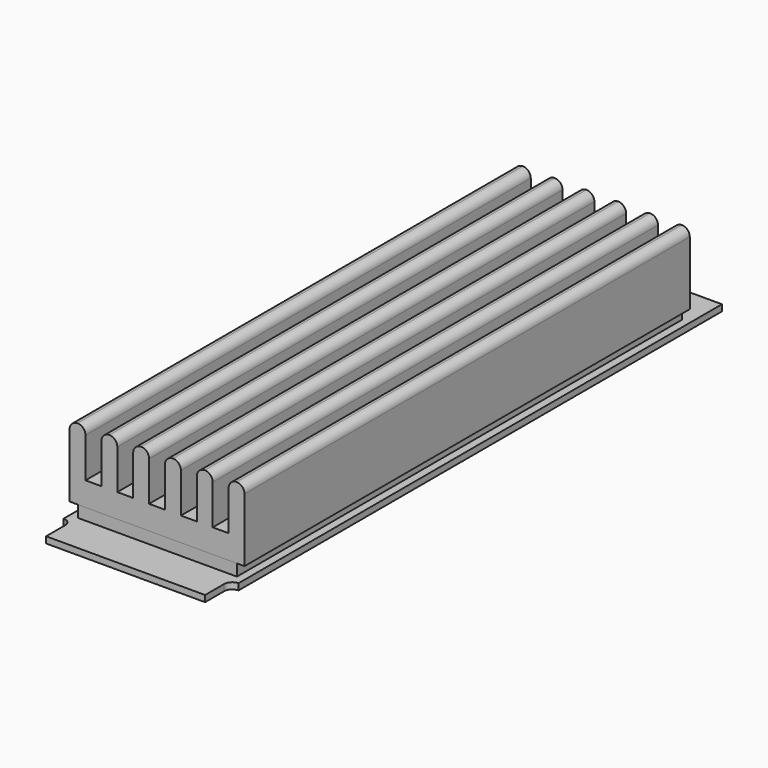
from build123d import *

# Parameters (mm, degrees)
F1_DEPTH = 0.8
F2_R     = 0.99999
F3_W     = 20
F3_H     = 70
F4_DEPTH = 1.5
F6_DEPTH = 0.801
F7_DEPTH = 0.1
F8_W     = 1
F8_H     = 2
F8_W_2   = 2
F8_H_2   = 6
F9_DEPTH = 35
F10_R    = 0.99999


# Not quite as in the source:
# - a fillet or chamfer is up to 0.001 mm smaller than in the source, because OpenCascade refuses the exact size


with BuildPart() as f1:
    # F0 (on Top) → F1 (new body)
    with BuildSketch(Plane.XY):
        Polygon((10.6782857925, 40.0528391576), (-11.3217142075, 40.0528391576), (-11.3217142075, -35.9471608424), (-10.3217142075, -35.9471608424), (-10.3217142075, -39.9471608424), (9.6782857925, -39.9471608424), (9.6782857925, -35.9471608424), (10.6782857925, -35.9471608424), align=None)
    extrude(amount=F1_DEPTH)

    # F2 (radius 1 in the source; OpenCascade refuses exactly that, so slightly less here)
    f2_edges = [f1.edges().sort_by_distance(p)[0] for p in [
        (9.678286, -35.947161, 0.4),
        (-10.321714, -35.947161, 0.4),
    ]]
    fillet(f2_edges, radius=F2_R)

    # F3 (on face) → F4 (join)
    with BuildSketch(Plane.XY.offset(0.8)):
        with Locations((-0.3217142075, 0.0528391576)):
            Rectangle(F3_W, F3_H)
    extrude(amount=F4_DEPTH)

    # F5 (on face) → F6 (cut, through all)
    with BuildSketch(Plane.XY.offset(0.8)):
        with BuildLine():
            ThreePointArc((-1.8217142075, 40.0528391576), (-0.3217142075, 38.5528391576), (1.1782857925, 40.0528391576))
            Line((1.1782857925, 40.0528391576), (-1.8217142075, 40.0528391576))
        make_face()
    extrude(amount=-F6_DEPTH, mode=Mode.SUBTRACT)

    # F5 (on face) → F7 (join)
    with BuildSketch(Plane.XY.offset(0.8)):
        with BuildLine():
            Line((2.4282857925, 40.0528391576), (1.1782857925, 40.0528391576))
            ThreePointArc((1.1782857925, 40.0528391576), (-0.3217142075, 38.5528391576), (-1.8217142075, 40.0528391576))
            Line((-1.8217142075, 40.0528391576), (-3.0717142075, 40.0528391576))
            ThreePointArc((-3.0717142075, 40.0528391576), (-0.3217142075, 37.3028391576), (2.4282857925, 40.0528391576))
        make_face()
    extrude(amount=F7_DEPTH)


with BuildPart() as f9:
    # F8 (on Front) → F9 (new body, symmetric)
    with BuildSketch(Plane.XZ):
        Polygon((-11.321724645, 3.3045688875), (-11.321724645, 2.3045688875), (10.678275355, 2.3045688875), (10.678275355, 3.3045688875), (9.678275355, 3.3045688875), (9.678275355, 5.3045688875), (8.678275355, 5.3045688875), (6.678275355, 5.3045688875), (4.678275355, 5.3045688875), (2.678275355, 5.3045688875), (0.678275355, 5.3045688875), (-1.321724645, 5.3045688875), (-3.321724645, 5.3045688875), (-5.321724645, 5.3045688875), (-7.321724645, 5.3045688875), (-9.321724645, 5.3045688875), (-10.321724645, 5.3045688875), (-10.321724645, 3.3045688875), align=None)
        with Locations((-10.821724645, 4.3045688875)):
            Rectangle(F8_W, F8_H)
        with Locations((10.178275355, 4.3045688875)):
            Rectangle(F8_W, F8_H)
        Polygon((-11.321724645, 11.3045688875), (-11.321724645, 5.3045688875), (-10.321724645, 5.3045688875), (-9.321724645, 5.3045688875), (-9.321724645, 11.3045688875), align=None)
        Polygon((9.678275355, 5.3045688875), (10.678275355, 5.3045688875), (10.678275355, 11.3045688875), (8.678275355, 11.3045688875), (8.678275355, 5.3045688875), align=None)
        with Locations((-6.321724645, 8.3045688875)):
            Rectangle(F8_W_2, F8_H_2)
        with Locations((5.678275355, 8.3045688875)):
            Rectangle(F8_W_2, F8_H_2)
        with Locations((-2.321724645, 8.3045688875)):
            Rectangle(F8_W_2, F8_H_2)
        with Locations((1.678275355, 8.3045688875)):
            Rectangle(F8_W_2, F8_H_2)
    extrude(amount=F9_DEPTH, both=True)

    # F10 (radius 1 in the source; OpenCascade refuses exactly that, so slightly less here)
    f10_edges = [f9.edges().sort_by_distance(p)[0] for p in [
        (-11.321725, 0, 11.304569),
        (-9.321725, 0, 11.304569),
        (-7.321725, 0, 11.304569),
        (-5.321725, 0, 11.304569),
        (-3.321725, 0, 11.304569),
        (-1.321725, 0, 11.304569),
        (0.678275, 0, 11.304569),
        (2.678275, 0, 11.304569),
        (4.678275, 0, 11.304569),
        (6.678275, 0, 11.304569),
        (8.678275, 0, 11.304569),
        (10.678275, 0, 11.304569),
    ]]
    fillet(f10_edges, radius=F10_R)


solid = Compound([f1.part, f9.part])
